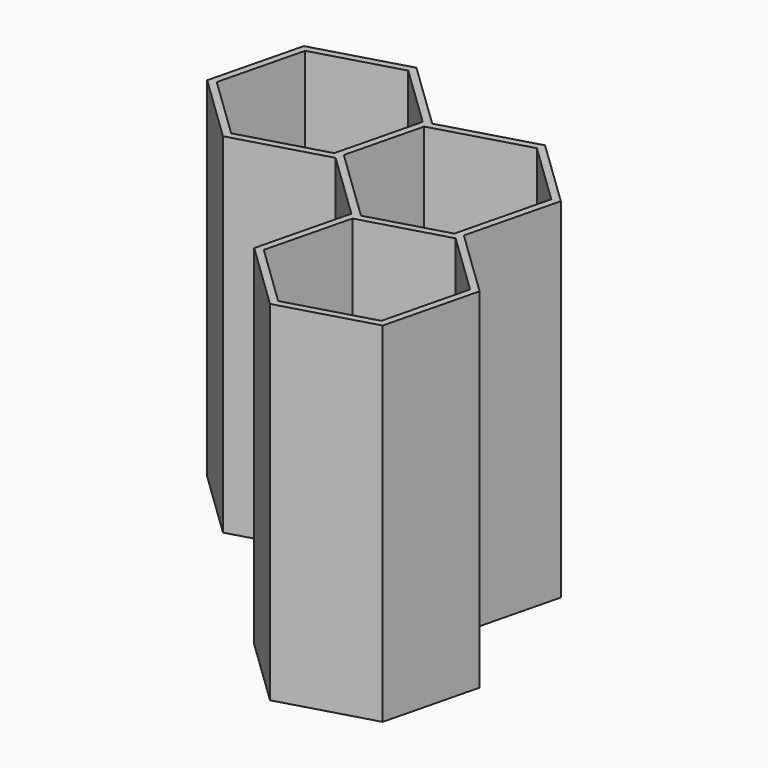
from build123d import *

# Parameters (mm, degrees)
F1_DEPTH = 2.5
F2_DEPTH = 100


with BuildPart() as f1:
    # F0 (on Top) → F1 (new body)
    with BuildSketch(Plane.XY):
        Polygon((23.9740391848, -53.6968420277), (47.9952290893, -46.7699065169), (54.0069219188, -22.503478075), (35.9974248438, -5.163985144), (11.9762349393, -12.0909206548), (5.9645421098, -36.3573490966), align=None)
    extrude(amount=F1_DEPTH)


with BuildPart() as f1b:
    # F0 (on Top) → F1, piece 2 (new body)
    with BuildSketch(Plane.XY):
        Polygon((12.5938805561, -9.8313160485), (34.3337787663, -3.5622313982), (40.9060056961, 22.9668144158), (22.9034034312, 40.2996690431), (-3.3346036331, 32.7334750457), (-8.7811057818, 10.7484604419), align=None)
    extrude(amount=F1_DEPTH)


with BuildPart() as f1c:
    # F0 (on Top) → F1, piece 3 (new body)
    with BuildSketch(Plane.XY):
        Polygon((-35.0032359624, 3.1868448251), (-11.0000882551, 10.1085775488), (-5.0077850981, 34.2967388346), (-23.0612686958, 51.6785818655), (-47.0666128749, 44.7562157503), (-53.0583663292, 20.5702733605), align=None)
    extrude(amount=F1_DEPTH)


with BuildPart() as f2:
    # F0 (on Top) → F2 (new body)
    with BuildSketch(Plane.XY):
        Polygon((56.225904392, -21.8635951819), (36.5527612395, -2.9223485051), (34.3337787663, -3.5622313982), (12.5938805561, -9.8313160485), (10.3748980829, -10.4711989416), (10.3125888618, -10.489166909), (3.7455596365, -36.9972319897), (23.418702789, -55.9384786666), (49.6588751668, -48.3716602627), align=None)
        Polygon((54.0069219188, -22.503478075), (47.9952290893, -46.7699065169), (23.9740391848, -53.6968420277), (5.9645421098, -36.3573490966), (11.9762349393, -12.0909206548), (35.9974248438, -5.163985144), align=None, mode=Mode.SUBTRACT)
        Polygon((34.3337787663, -3.5622313982), (36.5527612395, -2.9223485051), (43.1249881693, 23.6066973089), (23.458739827, 42.541305682), (-2.7792672374, 34.9751116846), (-2.7888026249, 34.9366217277), (-3.3346036331, 32.7334750457), (22.9034034312, 40.2996690431), (40.9060056961, 22.9668144158), align=None)
        Polygon((10.3748980829, -10.4711989416), (12.5938805561, -9.8313160485), (-8.7811057818, 10.7484604419), (-9.3364421776, 8.506823803), align=None)
        Polygon((-9.3364421776, 8.506823803), (-8.7811057818, 10.7484604419), (-3.3346036331, 32.7334750457), (-2.7888026249, 34.9366217277), (-22.5059323001, 53.9202185044), (-48.7302589523, 46.3579694961), (-55.2773488024, 19.9303904674), (-35.5585723582, 0.9452081862), align=None)
        Polygon((-5.0077850981, 34.2967388346), (-11.0000882551, 10.1085775488), (-35.0032359624, 3.1868448251), (-53.0583663292, 20.5702733605), (-47.0666128749, 44.7562157503), (-23.0612686958, 51.6785818655), align=None, mode=Mode.SUBTRACT)
    extrude(amount=F2_DEPTH)


solid = Compound([f1.part, f1b.part, f1c.part, f2.part])
